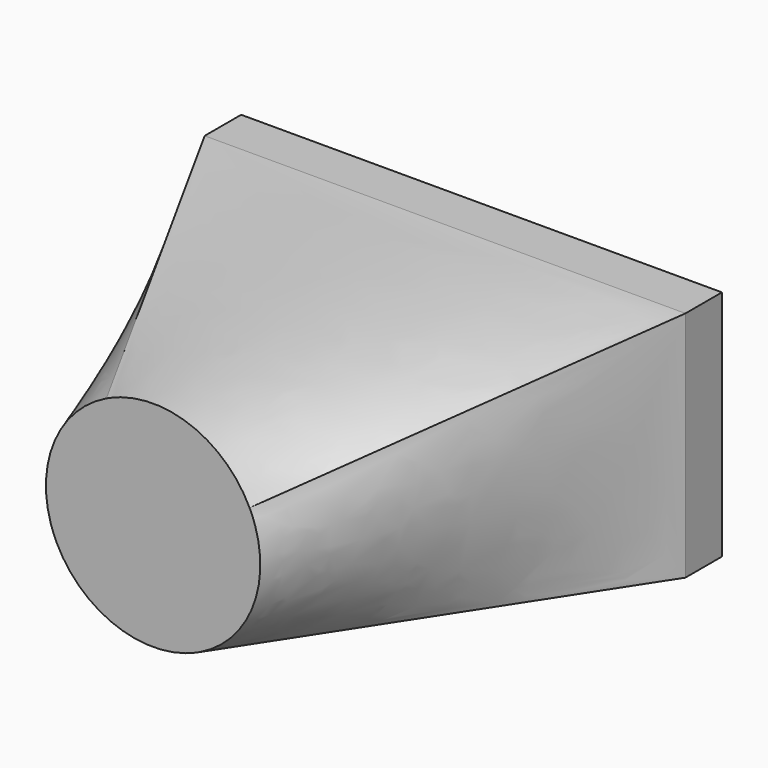
from build123d import *

# Parameters (mm, degrees)
F0_W     = 10.54
F0_H     = 5.1
F1_DEPTH = 1
F4_W     = 10.54
F4_H     = 5.1


# Not quite as in the source:
# - the arcs of a loft's sections are written as splines that run evenly, so that the points pair up as in the source's solid


with BuildPart() as f1:
    # F0 (on Front) → F1 (new body)
    with BuildSketch(Plane.XZ):
        Rectangle(F0_W, F0_H)
    extrude(amount=F1_DEPTH)

    # F3 (on offset) → F5 section 0
    with BuildSketch(Plane.XZ.offset(9)):
        with BuildLine():
            add(Edge.make_bspline(
                [(-2.1153742408, -1.023568181), (-1.9813894792, -1.3004700217), (-1.7923999056, -1.5506221732), (-1.3328968542, -1.9597225624), (-1.0625641713, -2.1185098365), (-0.4814827659, -2.320625108), (-0.1709626741, -2.3638735816), (0.4432327089, -2.3282335174), (0.7466663404, -2.2493590024), (1.023568181, -2.1153742408)],
                knots=[0, 0, 0, 0, 0.25, 0.25, 0.5, 0.5, 0.75, 0.75, 1, 1, 1, 1], degree=3))
            add(Edge.make_bspline(
                [(1.023568181, -2.1153742408), (1.3004700217, -1.9813894792), (1.5506221732, -1.7923999056), (1.9597225624, -1.3328968542), (2.1185098365, -1.0625641713), (2.320625108, -0.4814827659), (2.3638735816, -0.1709626741), (2.3282335174, 0.4432327089), (2.2493590024, 0.7466663404), (2.1153742408, 1.023568181)],
                knots=[0, 0, 0, 0, 0.25, 0.25, 0.5, 0.5, 0.75, 0.75, 1, 1, 1, 1], degree=3))
            add(Edge.make_bspline(
                [(2.1153742408, 1.023568181), (1.9813894792, 1.3004700217), (1.7923999056, 1.5506221732), (1.3328968542, 1.9597225624), (1.0625641713, 2.1185098365), (0.4814827659, 2.320625108), (0.1709626741, 2.3638735816), (-0.4432327089, 2.3282335174), (-0.7466663404, 2.2493590024), (-1.023568181, 2.1153742408)],
                knots=[0, 0, 0, 0, 0.25, 0.25, 0.5, 0.5, 0.75, 0.75, 1, 1, 1, 1], degree=3))
            add(Edge.make_bspline(
                [(-1.023568181, 2.1153742408), (-1.3004700217, 1.9813894792), (-1.5506221732, 1.7923999056), (-1.9597225624, 1.3328968542), (-2.1185098365, 1.0625641713), (-2.320625108, 0.4814827659), (-2.3638735816, 0.1709626741), (-2.3282335174, -0.4432327089), (-2.2493590024, -0.7466663404), (-2.1153742408, -1.023568181)],
                knots=[0, 0, 0, 0, 0.25, 0.25, 0.5, 0.5, 0.75, 0.75, 1, 1, 1, 1], degree=3))
        make_face()
    # F4 (on face) → F5 section 1
    with BuildSketch(Plane.XZ.offset(1)):
        Rectangle(F4_W, F4_H)
    loft(ruled=True)


solid = f1.part
